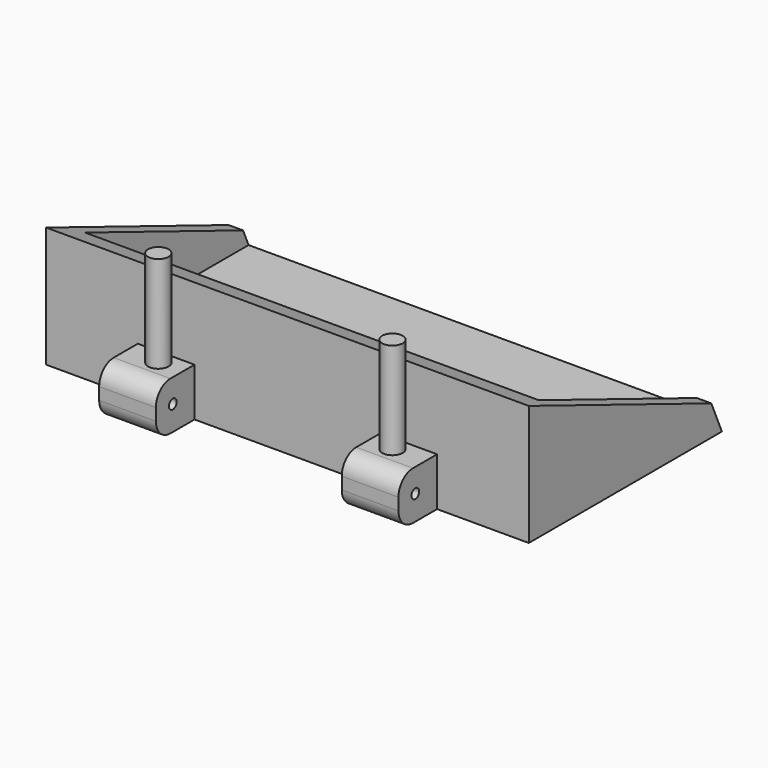
from build123d import *

# Parameters (mm, degrees)
F1_DEPTH = 50.8
F0_R     = 1.016
F2_DEPTH = 31.496
F3_R     = 2.159
F4_DEPTH = 20.32
F3_W     = 39.116
F3_H     = 6.35
F3_H_2   = 9.431579427
F5_DEPTH = 25.4
F6_W     = 95.504
F6_H     = 27.8849071284
F7_DEPTH = 35.56


with BuildPart() as f1:
    # F0 (on Right) → F1 (new body, symmetric)
    with BuildSketch(Plane.YZ):
        Polygon((-42.0039315899, 10.0997092374), (-35.6157857536, 10.0997092374), (8.7960684101, 10.0997092374), (6.0031614266, 16.4607279003), (-42.0039315899, 35.4997092374), (-42.0039315899, 20.2597092374), align=None)
    extrude(amount=F1_DEPTH, both=True)

    # F0 (on Right) → F2 (join, symmetric)
    with BuildSketch(Plane.YZ):
        with BuildLine():
            Line((-48.3539315899, 10.0997092374), (-42.0039315899, 10.0997092374))
            Line((-42.0039315899, 10.0997092374), (-42.0039315899, 20.2597092374))
            Line((-42.0039315899, 20.2597092374), (-48.3539315899, 20.2597092374))
            ThreePointArc((-48.3539315899, 20.2597092374), (-51.0480084262, 19.1437860737), (-52.1639315899, 16.4497092374))
            Line((-52.1639315899, 16.4497092374), (-52.1639315899, 13.9097092374))
            ThreePointArc((-52.1639315899, 13.9097092374), (-51.0480084262, 11.215632401), (-48.3539315899, 10.0997092374))
        make_face()
        with Locations((-47.7287806571, 15.2929993346)):
            Circle(F0_R, mode=Mode.SUBTRACT)
    extrude(amount=F2_DEPTH, both=True)

    # F3 (on face) → F4 (join)
    with BuildSketch(Plane.XY.offset(20.2597092374)):
        with Locations((-24.638, -45.1789315899)):
            Circle(F3_R)
        with Locations((24.638, -45.1789315899)):
            Circle(F3_R)
    extrude(amount=F4_DEPTH)

    # F3 (on face) → F5 (cut)
    with BuildSketch(Plane.XY.offset(20.2597092374)):
        with Locations((0, -45.1789315899)):
            Rectangle(F3_W, F3_H)
        with Locations((0, -53.0697213034)):
            Rectangle(F3_W, F3_H_2)
    extrude(amount=-F5_DEPTH, mode=Mode.SUBTRACT)

    # F6 (on Front) → F7 (cut, symmetric)
    with BuildSketch(Plane.XZ):
        with Locations((0, 27.0901628016)):
            Rectangle(F6_W, F6_H)
    extrude(amount=F7_DEPTH, both=True, mode=Mode.SUBTRACT)


solid = f1.part
